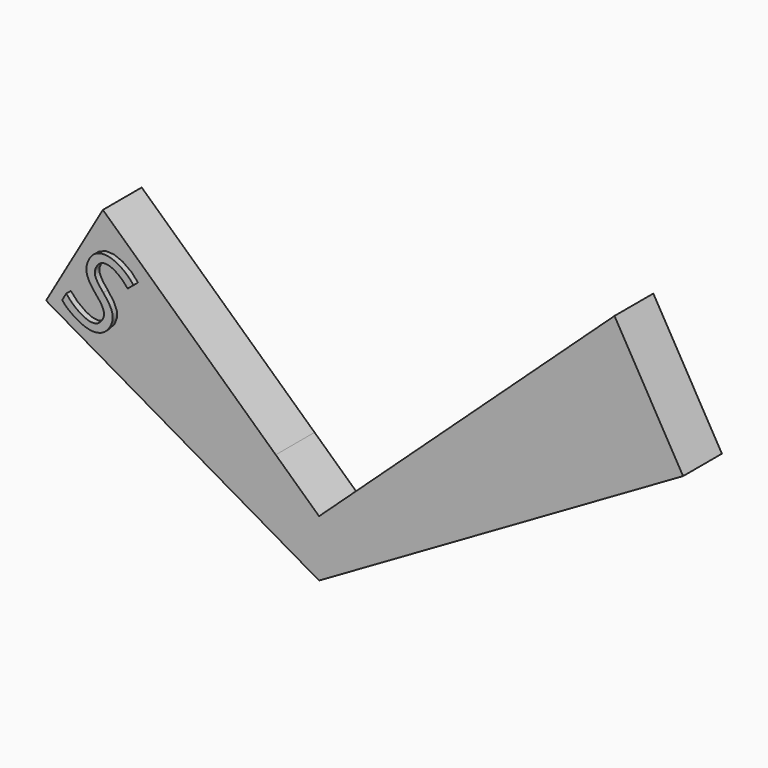
from build123d import *

# Parameters (mm, degrees)
F1_DEPTH     = 6
F2_TEXT_SIZE = 12.5
F3_DEPTH     = 2
F4_ANGLE     = 30


# Not quite as in the source:
# - a feature of the source that left no trace in its solid (it failed there, or was rolled back) is left out
# - Text() gives the source's letters only with a copy of the font that has no kerning and outlines rounded to 1/6400 em; it was checked with that copy


with BuildPart() as f1:
    # F0 (on Front) → F1 (new body)
    with BuildSketch(Plane.XZ):
        with BuildLine():
            Line((-33.7499343198, 15.9999620514), (-9.7675722182, 2.1434861705))
            ThreePointArc((-9.7675722182, 2.1434861705), (-8.1930408111, 5.7335924399), (-5.3594018945, 8.442559525))
            Line((-5.3594018945, 8.442559525), (-26.7295659142, 28.1505996764))
            Line((-26.7295659142, 28.1505996764), (-33.7499343198, 15.9999620514))
        make_face()
        with BuildLine():
            ThreePointArc((-5.3594018945, 8.442559525), (-8.1930408111, 5.7335924399), (-9.7675722182, 2.1434861705))
            Line((-9.7675722182, 2.1434861705), (0, -3.5))
            Line((0, -3.5), (0, 0))
            Line((0, 0), (0, 3.5))
            Line((0, 3.5), (-5.3594018945, 8.442559525))
        make_face()
        with BuildLine():
            ThreePointArc((5.3594018945, 8.442559525), (8.1930408111, 5.7335924399), (9.7675722182, 2.1434861705))
            Line((9.7675722182, 2.1434861705), (45, 22.5))
            Line((45, 22.5), (36.519007732, 37.1786404639))
            Line((36.519007732, 37.1786404639), (5.3594018945, 8.442559525))
        make_face()
        with BuildLine():
            Line((0, -3.5), (9.7675722182, 2.1434861705))
            ThreePointArc((9.7675722182, 2.1434861705), (8.1930408111, 5.7335924399), (5.3594018945, 8.442559525))
            Line((5.3594018945, 8.442559525), (0, 3.5))
            Line((0, 3.5), (0, 0))
            Line((0, 0), (0, -3.5))
        make_face()
    extrude(amount=F1_DEPTH)


with BuildPart() as f3:
    # F2 (on face) → F3 (new body)
    with BuildSketch(Plane.XZ.offset(6)):
        with Locations((-34.4394036133, 18.9711087109)):
            Text('S', F2_TEXT_SIZE, font='Open Sans', text_align=(TextAlign.LEFT, TextAlign.BOTTOM))
    extrude(amount=F3_DEPTH)


with BuildPart() as f3_1:
    # F4: moved
    add(f3.part.rotate(Axis((-26.7295659142, -3, 28.1505996764), (0, 1, 0)), F4_ANGLE))


with BuildPart() as f3_2:
    # F5: moved
    add(f3_1.part.moved(Location((6.1, 1.3, -6.8))))


solid = Compound([f1.part, f3_2.part])
